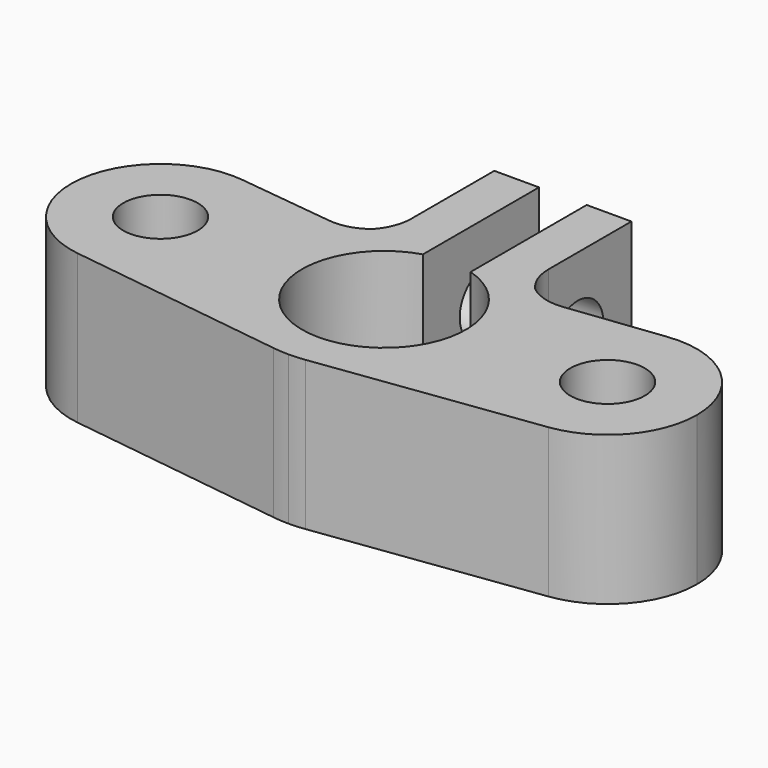
from build123d import *

# Parameters (mm, degrees)
F0_R        = 2.5
F1_DEPTH    = 10
F2_R        = 2.15
F3_DEPTH    = 25
F5_T1_DEPTH = 10


# Not quite as in the source:
# - a fillet or chamfer that OpenCascade refuses, or shapes differently, is made with other operations: its cross-section is extruded or revolved along the edge and cut away or added


with BuildPart() as f1:
    # F0 (on Top) → F1 (new body)
    with BuildSketch(Plane.XY):
        with BuildLine():
            ThreePointArc((1.6, 5.2621288468), (5.4402071954, -0.8087927246), (0, -5.5))
            Line((0, -5.5), (0, -8))
            ThreePointArc((0, -8), (0.5345278854, -7.982122521), (1.0666667681, -7.9285699849))
            ThreePointArc((1.0666667681, -7.9285699849), (7.426445373, -2.9745435149), (6.2449979984, 5))
            ThreePointArc((6.2449979984, 5), (5.477264575, 5.8309152605), (4.6, 6.5452272688))
            ThreePointArc((4.6, 6.5452272688), (3.166710076, 7.3465602355), (1.6, 7.8383671769))
            Line((1.6, 7.8383671769), (1.6, 5.2621288468))
        make_face()
        with BuildLine():
            ThreePointArc((6.2449979984, 5), (7.426445373, -2.9745435149), (1.0666667681, -7.9285699849))
            Line((1.0666667681, -7.9285699849), (15.8, -5.9464274989))
            ThreePointArc((15.8, -5.9464274989), (9.0476534506, -0.7546989834), (14.2906457894, 5.9579204932))
            Line((14.2906457894, 5.9579204932), (6.2449979984, 5))
        make_face()
        with BuildLine():
            Line((1.6, 15), (1.6, 7.8383671769))
            ThreePointArc((1.6, 7.8383671769), (3.166710076, 7.3465602355), (4.6, 6.5452272688))
            Line((4.6, 6.5452272688), (4.6, 15))
            Line((4.6, 15), (1.6, 15))
        make_face()
        with BuildLine():
            ThreePointArc((14.2906457894, 5.9579204932), (9.0476534506, -0.7546989834), (15.8, -5.9464274989))
            ThreePointArc((15.8, -5.9464274989), (19.5166359163, -3.9496835316), (21, 0))
            ThreePointArc((21, 0), (18.9839600109, 4.4864309458), (14.2906457894, 5.9579204932))
        make_face()
        with Locations((15, 0)):
            Circle(F0_R, mode=Mode.SUBTRACT)
    extrude(amount=F1_DEPTH)

    # F2 (on face) → F3 (cut)
    with BuildSketch(Plane.YZ.offset(4.6)):
        with Locations((10.5, 5)):
            Circle(F2_R)
    extrude(amount=-F3_DEPTH, mode=Mode.SUBTRACT)

    # F4: F1 across plane


with BuildPart() as f1_1:
    add(f1.part)
    add(f1.part.mirror(Plane.YZ))

    # F5: fillet of radius 3.2 on 4 edges, made by hand

    # F5_s2 → F5_t1 (join)
    with BuildSketch(Plane.XY):
        with BuildLine():
            ThreePointArc((-5.5714285714, 5.7410089421), (-4.8528464095, 6.790702563), (-4.6, 8.037412519))
            Line((-4.6, 8.037412519), (-4.6, 6.5452272688))
            ThreePointArc((-4.6, 6.5452272688), (-5.1015861823, 6.1622900309), (-5.5714285714, 5.7410089421))
        make_face()
        with BuildLine():
            ThreePointArc((-7.8251476511, 5.1881337307), (-6.4876416555, 5.3128293037), (-5.3191610039, 5.9754938051))
            ThreePointArc((-5.3191610039, 5.9754938051), (-5.8026149621, 5.5072370206), (-6.2449979984, 5))
            Line((-6.2449979984, 5), (-7.8251476511, 5.1881337307))
        make_face()
        with BuildLine():
            ThreePointArc((7.8251476511, 5.1881337307), (6.4876416555, 5.3128293037), (5.3191610039, 5.9754938051))
            ThreePointArc((5.3191610039, 5.9754938051), (5.8026149621, 5.5072370206), (6.2449979984, 5))
            Line((6.2449979984, 5), (7.8251476511, 5.1881337307))
        make_face()
        with BuildLine():
            ThreePointArc((5.5714285714, 5.7410089421), (4.8528464095, 6.790702563), (4.6, 8.037412519))
            Line((4.6, 8.037412519), (4.6, 6.5452272688))
            ThreePointArc((4.6, 6.5452272688), (5.1015861823, 6.1622900309), (5.5714285714, 5.7410089421))
        make_face()
    extrude(amount=F5_T1_DEPTH)


solid = f1_1.part
